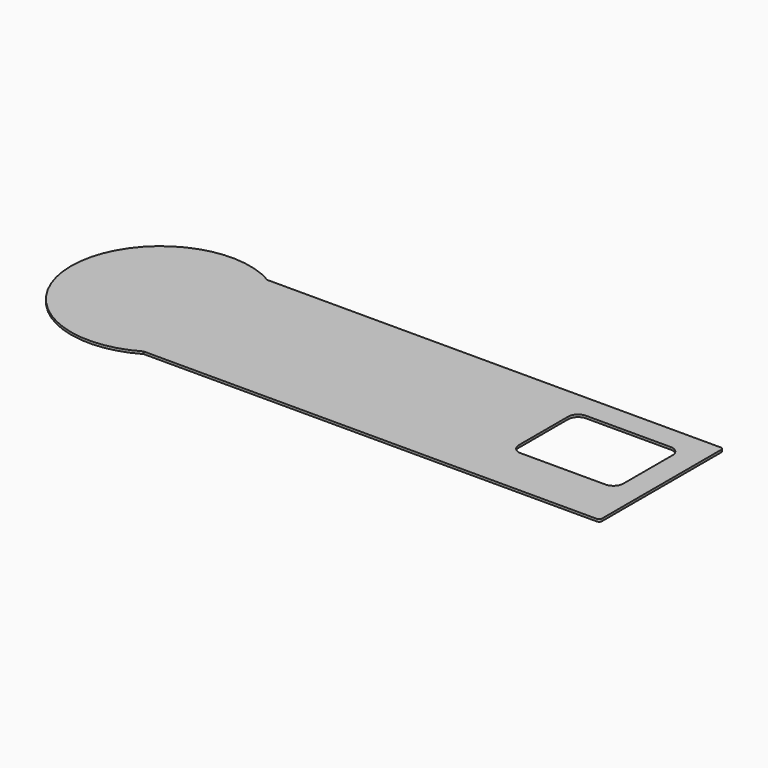
from build123d import *

# Parameters (mm, degrees)
F0_W     = 551.17
F0_H     = 155.58
F1_DEPTH = 2.38125
F2_R     = 3
F3_W     = 105
F3_H     = 81.79
F4_DEPTH = 25
F5_R     = 10
F6_R     = 90
F7_DEPTH = 2.38125


# Not quite as in the source:
# - a length typed as a fraction of an inch, garbled in the dataset ("3 / 203.2 mm" for 3/8 in), is restored


with BuildPart() as f1:
    # F0 (on Top) → F1 (new body)
    with BuildSketch(Plane.XY):
        Rectangle(F0_W, F0_H)
    extrude(amount=F1_DEPTH)

    # F2
    f2_edges = [f1.edges().sort_by_distance(p)[0] for p in [
        (275.585, -77.79, 1.190625),
        (-275.585, -77.79, 1.190625),
        (-275.585, 77.79, 1.190625),
        (275.585, 77.79, 1.190625),
    ]]
    fillet(f2_edges, radius=F2_R)

    # F3 (on face) → F4 (cut)
    with BuildSketch(Plane.XY.offset(2.38125)):
        with Locations((199.085, 12.895)):
            Rectangle(F3_W, F3_H)
    extrude(amount=-F4_DEPTH, mode=Mode.SUBTRACT)

    # F5
    f5_edges = [f1.edges().sort_by_distance(p)[0] for p in [
        (146.585, 53.79, 1.190625),
        (146.585, -28, 1.190625),
        (251.585, 53.79, 1.190625),
        (251.585, -28, 1.190625),
    ]]
    fillet(f5_edges, radius=F5_R)

    # F6 (on face) → F7 (join, through all)
    with BuildSketch(Plane.XY.offset(2.38125)):
        with Locations((-228.1388989337, 0)):
            Circle(F6_R)
    extrude(amount=-F7_DEPTH)


solid = f1.part
